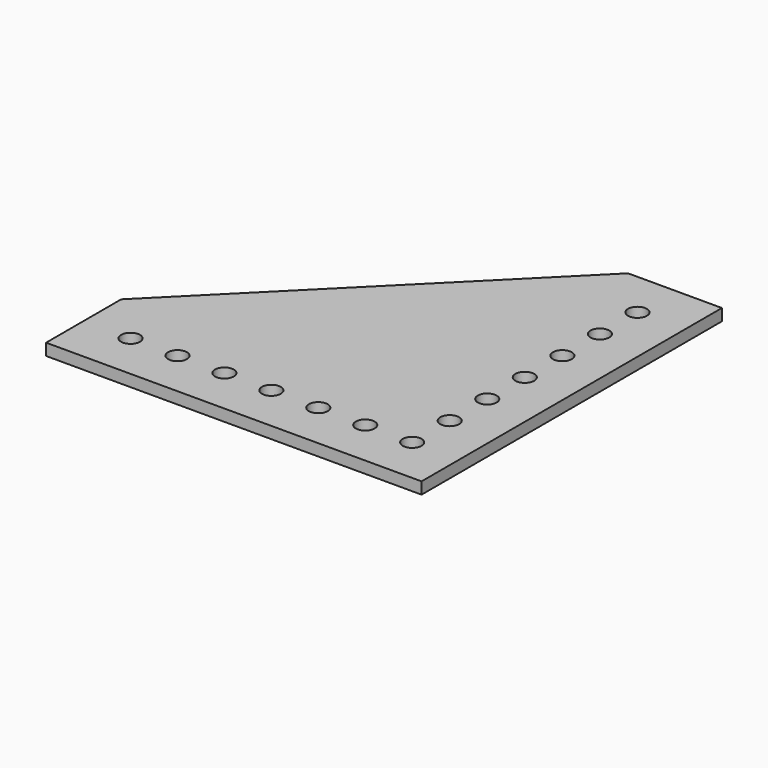
from build123d import *

# Parameters (mm, degrees)
F0_R     = 2.5527
F1_DEPTH = 3.175


# Not quite as in the source:
# - a length typed as a fraction of an inch, garbled in the dataset ("3 / 203.2 mm" for 3/8 in), is restored


with BuildPart() as f1:
    # F0 (on Top) → F1 (new body)
    with BuildSketch(Plane.XY):
        Polygon((0, 25.4), (0, 0), (101.6, 0), (101.6, 101.6), (76.2, 101.6), (76.2, 25.4), align=None)
        with Locations((12.7, 12.7)):
            Circle(F0_R, mode=Mode.SUBTRACT)
        with Locations((25.4, 12.7)):
            Circle(F0_R, mode=Mode.SUBTRACT)
        with Locations((38.1, 12.7)):
            Circle(F0_R, mode=Mode.SUBTRACT)
        with Locations((50.8, 12.7)):
            Circle(F0_R, mode=Mode.SUBTRACT)
        with Locations((63.5, 12.7)):
            Circle(F0_R, mode=Mode.SUBTRACT)
        with Locations((76.2, 12.7)):
            Circle(F0_R, mode=Mode.SUBTRACT)
        with Locations((88.9, 12.7)):
            Circle(F0_R, mode=Mode.SUBTRACT)
        with Locations((88.9, 25.4)):
            Circle(F0_R, mode=Mode.SUBTRACT)
        with Locations((88.9, 38.1)):
            Circle(F0_R, mode=Mode.SUBTRACT)
        with Locations((88.9, 50.8)):
            Circle(F0_R, mode=Mode.SUBTRACT)
        with Locations((88.9, 63.5)):
            Circle(F0_R, mode=Mode.SUBTRACT)
        with Locations((88.9, 76.2)):
            Circle(F0_R, mode=Mode.SUBTRACT)
        with Locations((88.9, 88.9)):
            Circle(F0_R, mode=Mode.SUBTRACT)
        Polygon((76.2, 101.6), (0, 25.4), (76.2, 25.4), align=None)
    extrude(amount=F1_DEPTH)


solid = f1.part
